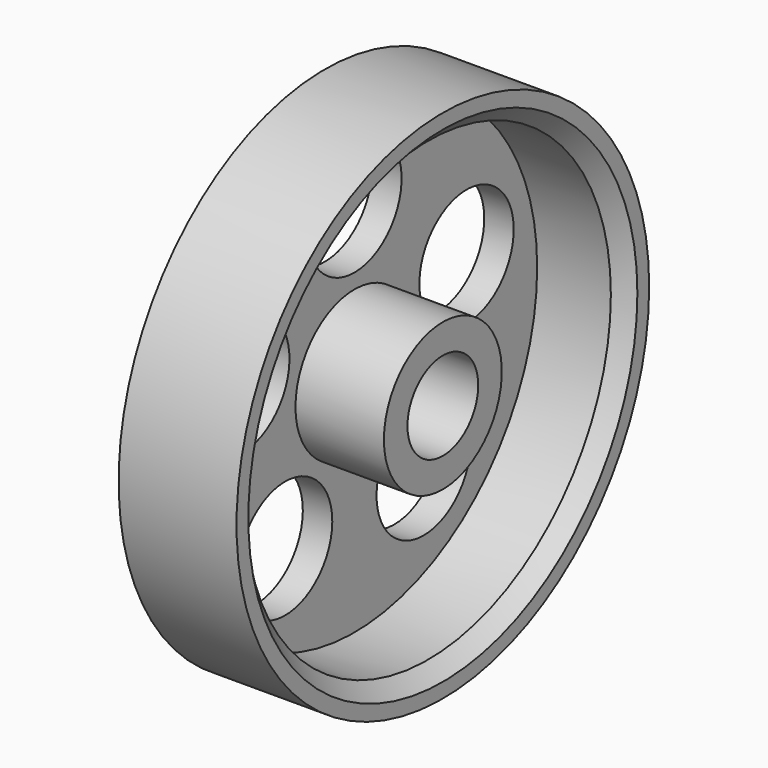
from build123d import *

# Parameters (mm, degrees)
F0_W            = 8
F0_H            = 17.5
F3_D            = 6
F4_T            = -2
F6_D            = 8
F6_COPIES_COUNT = 5
F7_SIZE         = 1


# Not quite as in the source:
# - a pattern or mirror of a feature is missing from the dataset's text; its kind, count and spacing are read off the source's solid


with BuildPart() as f1:
    # F0 (on Top) → F1 (revolve)
    with BuildSketch(Plane.XY):
        with Locations((4, 8.75)):
            Rectangle(F0_W, F0_H)
    revolve(axis=Axis((4, 0, 0), (1, 0, 0)))

    # F3 (through all)
    with Locations(Plane(origin=(0, 0, 0), x_dir=(0, 1, 0), z_dir=(-1, 0, 0))):
        with Locations((0, 0)):
            Hole(F3_D / 2)

    # F4
    f4_openings = [f1.faces().sort_by_distance(p)[0] for p in [
        (8, -17.005025, 0),
    ]]
    offset(amount=F4_T, openings=f4_openings)

    # F6 (through all)
    with Locations(Plane(origin=(0, 0, 0), x_dir=(0, 1, 0), z_dir=(-1, 0, 0))):
        with Locations((0, -10)):
            f6 = Hole(F6_D / 2)

    # F6_copies: F6 ×5 about axis
    f6_copies_axis = Axis((0, 0, 0), (1, 0, 0))
    for i in range(1, F6_COPIES_COUNT):
        add(f6.rotate(f6_copies_axis, i * 360 / F6_COPIES_COUNT), mode=Mode.SUBTRACT)

    # F7
    f7_edges = [f1.edges().sort_by_distance(p)[0] for p in [
        (8, -15.5, 0),
    ]]
    chamfer(f7_edges, length=F7_SIZE)


solid = f1.part
